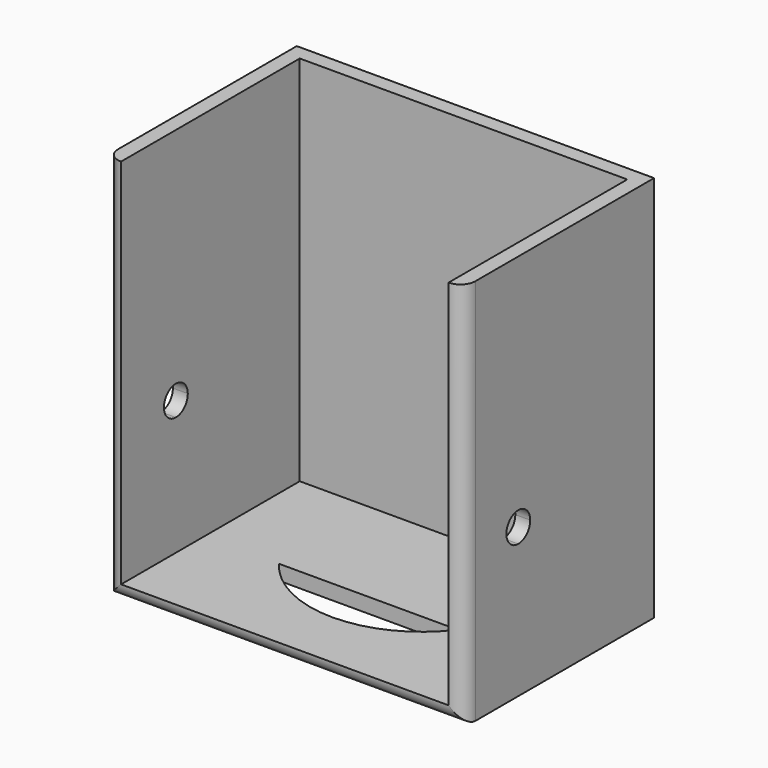
from build123d import *

# Parameters (mm, degrees)
F1_DEPTH      = 5
F2_DEPTH      = 125
F4_DEPTH      = 25
F4_DEPTH_BACK = 129
F5_W          = 60
F5_H          = 5
F6_DEPTH      = 10
F7_W          = 60
F7_H          = 5
F8_DEPTH      = 54
F9_R          = 4.99999
F11_DEPTH     = 64


# Not quite as in the source:
# - a fillet or chamfer is up to 0.001 mm smaller than in the source, because OpenCascade refuses the exact size
# - ends of sketch curves that miss each other by under 0.0002 mm in the source are joined


with BuildPart() as f1:
    # F0 (on Top) → F1 (new body)
    with BuildSketch(Plane.XY):
        Polygon((55, -40), (60, -40), (60, 40), (-60, 40), (-60, -40), (-55, -40), (-55, 35), (0, 35), (55, 35), align=None)
        with BuildLine():
            Line((-55, -40), (0, -40))
            Line((0, -40), (0, -20))
            ThreePointArc((0, -20), (-16.7705098312, -16.0410196625), (-30, -5))
            Line((-30, -5), (0, -5))
            Line((0, -5), (0, 35))
            Line((0, 35), (-55, 35))
            Line((-55, 35), (-55, -40))
        make_face()
        with BuildLine():
            Line((0, -40), (55, -40))
            Line((55, -40), (55, 35))
            Line((55, 35), (0, 35))
            Line((0, 35), (0, -5))
            Line((0, -5), (30, -5))
            ThreePointArc((30, -5), (16.7705098312, -16.0410196625), (0, -20))
            Line((0, -20), (0, -40))
        make_face()
    extrude(amount=-F1_DEPTH)

    # F0 (on Top) → F2 (join)
    with BuildSketch(Plane.XY):
        Polygon((55, -40), (60, -40), (60, 40), (-60, 40), (-60, -40), (-55, -40), (-55, 35), (0, 35), (55, 35), align=None)
    extrude(amount=F2_DEPTH)

    # F3 (on face) → F4 (cut, two sides)
    with BuildSketch(Plane.YZ.offset(-55)) as f4_sk:
        with BuildLine():
            Line((-17, 45), (-17, 40))
            ThreePointArc((-17, 40), (-13.4644660941, 41.4644660941), (-12, 45))
            Line((-12, 45), (-17, 45))
        make_face()
        with BuildLine():
            ThreePointArc((-12, 45), (-20.5355339059, 48.5355339059), (-17, 40))
            Line((-17, 40), (-17, 45))
            Line((-17, 45), (-12, 45))
        make_face()
    extrude(amount=-F4_DEPTH, mode=Mode.SUBTRACT)
    extrude(f4_sk.sketch, amount=F4_DEPTH_BACK, mode=Mode.SUBTRACT)

    # F5 (on face) → F6 (join)
    with BuildSketch(Plane(origin=(0, 40, 0), x_dir=(-1, 0, 0), z_dir=(0, 1, 0))):
        Polygon((30, 115), (0, 115), (-30, 115), (-30, 110), (30, 110), align=None)
        with Locations((0, 53.5)):
            Rectangle(F5_W, F5_H)
    extrude(amount=F6_DEPTH)

    # F7 (on face) → F8 (join, through all)
    with BuildSketch(Plane(origin=(0, 0, 110), x_dir=(1, 0, 0), z_dir=(0, 0, -1))):
        with Locations((0, -47.5)):
            Rectangle(F7_W, F7_H)
    extrude(amount=F8_DEPTH)

    # F9 (radius 5 in the source; OpenCascade refuses exactly that, so slightly less here)
    f9_edges = [f1.edges().sort_by_distance(p)[0] for p in [
        (-60, -40, 60),
        (0, -40, -5),
        (60, -40, 60),
        (-30, 50, 83),
        (30, 50, 83),
    ]]
    fillet(f9_edges, radius=F9_R)

    # F10 (on face) → F11 (join, through all)
    with BuildSketch(Plane.XY.offset(115)):
        with BuildLine():
            ThreePointArc((-17.5, 54), (-21.75, 52.9375), (-25, 50))
            Line((-25, 50), (-17.5, 50))
            Line((-17.5, 50), (-17.5, 54))
        make_face()
        with BuildLine():
            Line((-17.5, 54), (-17.5, 50))
            Line((-17.5, 50), (-10, 50))
            ThreePointArc((-10, 50), (-13.25, 52.9375), (-17.5, 54))
        make_face()
        with BuildLine():
            ThreePointArc((25, 50), (17.5, 54), (10, 50))
            Line((10, 50), (25, 50))
        make_face()
    extrude(amount=-F11_DEPTH)


solid = f1.part
